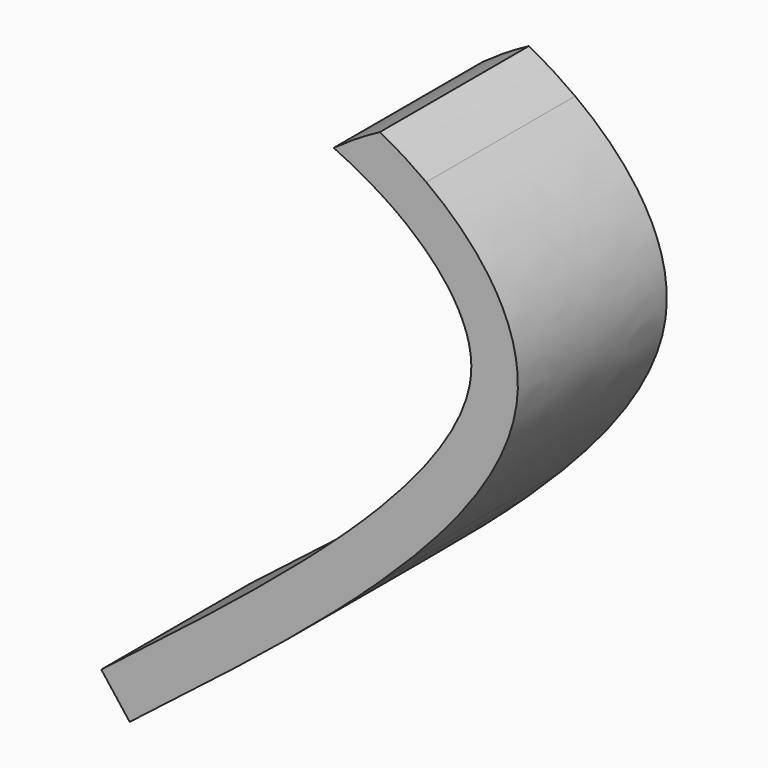
from build123d import *

# Parameters (mm, degrees)
F1_DEPTH = 25.4


# Not quite as in the source:
# - the dataset's text gives a spline's control points without its knots; the knots are read off the source's solid


with BuildPart() as f1:
    # F0 (on Front) → F1 (new body)
    with BuildSketch(Plane.XZ):
        with BuildLine():
            add(Edge.make_bspline(
                [(-34.1506078839, -55.8828152716), (-21.8914852414, -46.4478308529), (-9.6323625988, -37.0128464341), (0, -27.9183218871)],
                knots=[0, 0, 0, 0, 0.1514507337, 0.1514507337, 0.1514507337, 0.1514507337], degree=3))
            add(Edge.make_bspline(
                [(0, -27.9183218871), (-1.5842627041, -26.4225189723), (-3.0974680344, -24.9359259526), (-4.5279289777, -23.4600576062)],
                knots=[0.1514507337, 0.1514507337, 0.1514507337, 0.1514507337, 0.1763602766, 0.1763602766, 0.1763602766, 0.1763602766], degree=3))
            add(Edge.make_bspline(
                [(-38.0235321895, -50.8506231724), (-32.964493212, -46.9570367129), (-25.411988601, -41.1438409195), (-15.9773889577, -33.532464644), (-9.7671383953, -28.2635561204), (-6.0968542737, -24.9371703328), (-4.5279289777, -23.4600576062)],
                knots=[0, 0, 0, 0, 0.0625, 0.09375, 0.125, 0.1505345708, 0.1505345708, 0.1505345708, 0.1505345708], degree=3))
            Line((-38.0235321895, -50.8506231724), (-34.1506078839, -55.8828152716))
        make_face()
        with BuildLine():
            add(Edge.make_bspline(
                [(0, -27.9183218871), (-1.5842627041, -26.4225189723), (-3.0974680344, -24.9359259526), (-4.5279289777, -23.4600576062)],
                knots=[0.1514507337, 0.1514507337, 0.1514507337, 0.1514507337, 0.1763602766, 0.1763602766, 0.1763602766, 0.1763602766], degree=3))
            add(Edge.make_bspline(
                [(0, -27.9183218871), (1.5842627041, -26.4225189723), (3.0974680344, -24.9359259526), (4.5279289777, -23.4600576062)],
                knots=[0.1514507337, 0.1514507337, 0.1514507337, 0.1514507337, 0.1763602766, 0.1763602766, 0.1763602766, 0.1763602766], degree=3))
            add(Edge.make_bspline(
                [(4.5279289777, -23.4600576062), (4.176754816, -23.1294339463), (2.5965612537, -21.628469419), (1.1041846652, -20.1478487693), (0, -19.0077495537)],
                knots=[0.1505345708, 0.1505345708, 0.1505345708, 0.1505345708, 0.15625, 0.1765551098, 0.1765551098, 0.1765551098, 0.1765551098], degree=3))
            add(Edge.make_bspline(
                [(-4.5279289777, -23.4600576062), (-4.176754816, -23.1294339463), (-2.5965612537, -21.628469419), (-1.1041846652, -20.1478487693), (0, -19.0077495537)],
                knots=[0.1505345708, 0.1505345708, 0.1505345708, 0.1505345708, 0.15625, 0.1765551098, 0.1765551098, 0.1765551098, 0.1765551098], degree=3))
        make_face()
        with BuildLine():
            add(Edge.make_bspline(
                [(4.5279289777, -23.4600576062), (4.176754816, -23.1294339463), (2.5965612537, -21.628469419), (1.1041846652, -20.1478487693), (0, -19.0077495537)],
                knots=[0.1505345708, 0.1505345708, 0.1505345708, 0.1505345708, 0.15625, 0.1765551098, 0.1765551098, 0.1765551098, 0.1765551098], degree=3))
            add(Edge.make_bspline(
                [(4.5279289777, -23.4600576062), (12.5168165781, -15.2175771756), (24.2667467967, 1.9638440983), (14.2239104506, 16.3206592469), (6.3155328924, 22.1220430357)],
                knots=[0.1763602766, 0.1763602766, 0.1763602766, 0.1763602766, 0.3154759505, 0.4786127939, 0.4786127939, 0.4786127939, 0.4786127939], degree=3))
            add(Edge.make_bspline(
                [(0, 18.7410253917), (0.0872787473, 18.7959999139), (0.8887457213, 19.2970922185), (2.0827351169, 19.9945059246), (3.5997889629, 20.8032306784), (4.8816198644, 21.4479503665), (5.797109485, 21.8824591333), (6.3155328924, 22.1220430356)],
                knots=[0.498083134, 0.498083134, 0.498083134, 0.498083134, 0.5, 0.515625, 0.5234375, 0.53125, 0.5411756418, 0.5411756418, 0.5411756418, 0.5411756418], degree=3))
            add(Edge.make_bspline(
                [(0, -19.0077495537), (0.595179246, -18.3932115939), (2.8220785447, -16.0411764836), (6.2163099197, -12.0740204289), (8.945591137, -8.1335030302), (10.5463399287, -5.2209039688), (11.4515036009, -3.1786229516), (11.9634338293, -1.6123544417), (12.2364169712, -0.4465465374), (12.3762454919, 0.3846596029), (12.454803462, 1.174450343), (12.4862502571, 2.2150773983), (12.3928224576, 3.4949316017), (12.0736867403, 5.0344674335), (11.5414003406, 6.5964904077), (10.7881903271, 8.1853122273), (9.4849093503, 10.3288103404), (7.2993639863, 13.018534193), (4.4490347488, 15.6025237735), (1.9268617559, 17.4827420786), (0.6241588031, 18.3478846439), (0, 18.7410253917)],
                knots=[0.1765551098, 0.1765551098, 0.1765551098, 0.1765551098, 0.1875, 0.21875, 0.25, 0.265625, 0.28125, 0.296875, 0.3046875, 0.3125, 0.3203125, 0.328125, 0.34375, 0.359375, 0.375, 0.390625, 0.40625, 0.4375, 0.46875, 0.484375, 0.498083134, 0.498083134, 0.498083134, 0.498083134], degree=3))
        make_face()
        with BuildLine():
            add(Edge.make_bspline(
                [(-6.3155328924, 22.1220430357), (-4.3449197911, 23.5676344753), (-2.219831491, 24.8923026842), (0, 26.0786470026)],
                knots=[0.4786127939, 0.4786127939, 0.4786127939, 0.4786127939, 0.5192633064, 0.5192633064, 0.5192633064, 0.5192633064], degree=3))
            add(Edge.make_bspline(
                [(0, 18.7410253917), (-0.0872787473, 18.7959999139), (-0.8887457213, 19.2970922185), (-2.0827351169, 19.9945059246), (-3.5997889629, 20.8032306784), (-4.8816198644, 21.4479503665), (-5.797109485, 21.8824591333), (-6.3155328924, 22.1220430356)],
                knots=[0.498083134, 0.498083134, 0.498083134, 0.498083134, 0.5, 0.515625, 0.5234375, 0.53125, 0.5411756418, 0.5411756418, 0.5411756418, 0.5411756418], degree=3))
            add(Edge.make_bspline(
                [(0, 18.7410253917), (0.0872787473, 18.7959999139), (0.8887457213, 19.2970922185), (2.0827351169, 19.9945059246), (3.5997889629, 20.8032306784), (4.8816198644, 21.4479503665), (5.797109485, 21.8824591333), (6.3155328924, 22.1220430356)],
                knots=[0.498083134, 0.498083134, 0.498083134, 0.498083134, 0.5, 0.515625, 0.5234375, 0.53125, 0.5411756418, 0.5411756418, 0.5411756418, 0.5411756418], degree=3))
            add(Edge.make_bspline(
                [(6.3155328924, 22.1220430357), (4.3449197911, 23.5676344753), (2.219831491, 24.8923026842), (0, 26.0786470026)],
                knots=[0.4786127939, 0.4786127939, 0.4786127939, 0.4786127939, 0.5192633064, 0.5192633064, 0.5192633064, 0.5192633064], degree=3))
        make_face()
    extrude(amount=F1_DEPTH)


solid = f1.part
